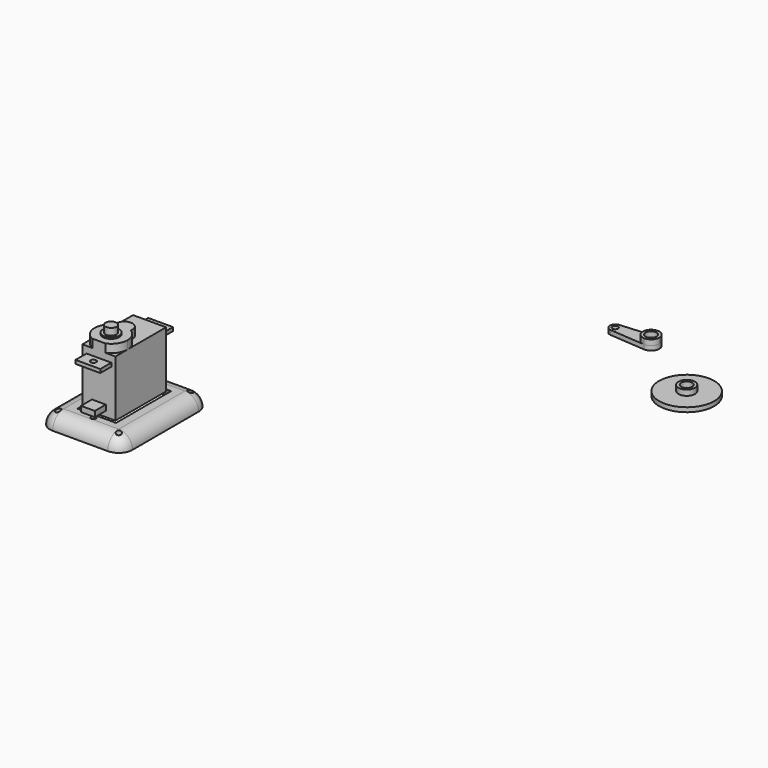
from build123d import *

# Parameters (mm, degrees)
F0_W          = 12
F0_H          = 23
F1_DEPTH      = 20.5
F3_DEPTH      = 3
F4_R          = 3
F5_DEPTH      = 0.5
F6_R          = 2
F7_DEPTH      = 2.5
F9_W          = 9
F9_H          = 5
F9_R          = 1
F10_DEPTH     = 1.3
F11_W         = 5
F11_H         = 2
F12_DEPTH     = 5
F13_R         = 10
F13_R_2       = 2.5
F14_DEPTH     = 0.5
F15_R         = 10
F15_R_2       = 2.5
F15_R_3       = 1
F16_DEPTH     = 1.1
F17_R         = 3
F17_R_2       = 2
F18_DEPTH     = 2
F19_R         = 2.5
F20_DEPTH     = 0.5
F22_R         = 2.5
F22_R_2       = 1
F21_R         = 2.5
F23_DEPTH     = 1.1
F24_R         = 2
F25_DEPTH     = 2
F26_R         = 1.05
F27_DEPTH     = 1.601
F28_W         = 30
F28_H         = 40
F28_R         = 0.9
F28_W_2       = 14
F28_H_2       = 25
F29_DEPTH     = 5
F30_T1_DEPTH  = 20
F30_T3_DEPTH  = 30
F30_T5_DEPTH  = 12.5
F30_S9_W      = 5
F30_S9_H      = 5
F30_T10_DEPTH = 5
F30_S15_W     = 5
F30_S15_H     = 5
F30_T16_DEPTH = 5
F30_S21_W     = 5
F30_S21_H     = 5
F30_T22_DEPTH = 5
F30_S27_W     = 5
F30_S27_H     = 5
F30_T28_DEPTH = 5
F31_T1_DEPTH  = 14


# Not quite as in the source:
# - a fillet or chamfer that OpenCascade refuses, or shapes differently, is made with other operations: its cross-section is extruded or revolved along the edge and cut away or added


with BuildPart() as f1:
    # F0 (on Top) → F1 (new body)
    with BuildSketch(Plane.XY):
        with Locations((-56.6354888082, -51.4608333111)):
            Rectangle(F0_W, F0_H)
    extrude(amount=F1_DEPTH)

    # F2 (on face) → F3 (join)
    with BuildSketch(Plane.XY.offset(20.5)):
        with BuildLine():
            ThreePointArc((-54.2375730465, -62.9608333111), (-51.6161514729, -60.7481198388), (-50.6354888082, -57.4608333111))
            ThreePointArc((-50.6354888082, -57.4608333111), (-51.4669094551, -54.4135743016), (-53.7307512985, -52.2108333111))
            ThreePointArc((-53.7307512985, -52.2108333111), (-56.6354888082, -51.4608333111), (-59.5402263178, -52.2108333111))
            ThreePointArc((-59.5402263178, -52.2108333111), (-61.8040681612, -54.4135743016), (-62.6354888082, -57.4608333111))
            ThreePointArc((-62.6354888082, -57.4608333111), (-61.6548261434, -60.7481198388), (-59.0334045698, -62.9608333111))
            Line((-59.0334045698, -62.9608333111), (-54.2375730465, -62.9608333111))
        make_face()
        with BuildLine():
            ThreePointArc((-59.5402263178, -52.2108333111), (-56.6354888082, -51.4608333111), (-53.7307512985, -52.2108333111))
            ThreePointArc((-53.7307512985, -52.2108333111), (-56.6354888082, -48.4608333111), (-59.5402263178, -52.2108333111))
        make_face()
    extrude(amount=F3_DEPTH)

    # F4 (on face) → F5 (join)
    with BuildSketch(Plane.XY.offset(23.5)):
        with Locations((-56.6354888082, -57.4608333111)):
            Circle(F4_R)
    extrude(amount=F5_DEPTH)

    # F6 (on face) → F7 (join)
    with BuildSketch(Plane.XY.offset(24)):
        with Locations((-56.6354888082, -57.4608333111)):
            Circle(F6_R)
    extrude(amount=F7_DEPTH)

    # F9 (on offset) → F10 (join)
    with BuildSketch(Plane.XY.offset(16.75)):
        with Locations((-56.6354888082, -65.4608333111)):
            Rectangle(F9_W, F9_H)
        with Locations((-56.6354888082, -65.4608333111)):
            Circle(F9_R, mode=Mode.SUBTRACT)
        with Locations((-56.6354888082, -37.4608333111)):
            Rectangle(F9_W, F9_H)
        with Locations((-56.6354888082, -37.4608333111)):
            Circle(F9_R, mode=Mode.SUBTRACT)
    extrude(amount=F10_DEPTH)

    # F11 (on face) → F12 (join, through all)
    with BuildSketch(Plane.XZ.offset(62.9608333111)):
        with Locations((-56.6354888082, 3)):
            Rectangle(F11_W, F11_H)
    extrude(amount=F12_DEPTH)


with BuildPart() as f14:
    # F13 (on Top) → F14 (new body)
    with BuildSketch(Plane.XY):
        with Locations((66.4411634207, 50.0796362758)):
            Circle(F13_R)
        with Locations((66.4411634207, 50.0796362758)):
            Circle(F13_R_2, mode=Mode.SUBTRACT)
    extrude(amount=F14_DEPTH)

    # F15 (on face) → F16 (join)
    with BuildSketch(Plane.XY.offset(0.5)):
        with Locations((66.4411634207, 50.0796362758)):
            Circle(F15_R)
        with Locations((66.4411634207, 50.0796362758)):
            Circle(F15_R_2, mode=Mode.SUBTRACT)
        with Locations((66.4411634207, 50.0796362758)):
            Circle(F15_R_2)
        with Locations((66.4411634207, 50.0796362758)):
            Circle(F15_R_3, mode=Mode.SUBTRACT)
    extrude(amount=F16_DEPTH)

    # F17 (on face) → F18 (join)
    with BuildSketch(Plane.XY.offset(1.6)):
        with Locations((66.4411634207, 50.0796362758)):
            Circle(F17_R)
        with Locations((66.4411634207, 50.0796362758)):
            Circle(F17_R_2, mode=Mode.SUBTRACT)
    extrude(amount=F18_DEPTH)


with BuildPart() as f20:
    # F19 (on Top) → F20 (new body)
    with BuildSketch(Plane.XY):
        with BuildLine():
            Line((26.1375896391, 65.84841691), (39.0606665622, 64.8513798795))
            ThreePointArc((39.0606665622, 64.8513798795), (42.291435793, 67.8424909711), (39.0606665622, 70.8336020627))
            Line((39.0606665622, 70.8336020627), (26.1375896391, 69.8365650321))
            ThreePointArc((26.1375896391, 69.8365650321), (24.291435793, 67.8424909711), (26.1375896391, 65.84841691))
        make_face()
        with Locations((39.291435793, 67.8424909711)):
            Circle(F19_R, mode=Mode.SUBTRACT)
    extrude(amount=F20_DEPTH)

    # F22 (on face) + F21 (on face) → F23 (join)
    with BuildSketch(Plane.XY.offset(0.5)):
        with Locations((39.291435793, 67.8424909711)):
            Circle(F22_R)
        with Locations((39.291435793, 67.8424909711)):
            Circle(F22_R_2, mode=Mode.SUBTRACT)
    with BuildSketch(Plane.XY.offset(0.5)):
        with BuildLine():
            ThreePointArc((39.0606665622, 64.8513798795), (42.291435793, 67.8424909711), (39.0606665622, 70.8336020627))
            Line((39.0606665622, 70.8336020627), (26.1375896391, 69.8365650321))
            ThreePointArc((26.1375896391, 69.8365650321), (24.291435793, 67.8424909711), (26.1375896391, 65.84841691))
            Line((26.1375896391, 65.84841691), (39.0606665622, 64.8513798795))
        make_face()
        with Locations((39.291435793, 67.8424909711)):
            Circle(F21_R, mode=Mode.SUBTRACT)
    extrude(amount=F23_DEPTH)

    # F24 (on face) → F25 (join)
    with BuildSketch(Plane.XY.offset(1.6)):
        with BuildLine():
            ThreePointArc((39.0606665622, 64.8513798795), (41.3295344544, 65.641092814), (42.291435793, 67.8424909711))
            ThreePointArc((42.291435793, 67.8424909711), (41.3295344544, 70.0438891282), (39.0606665622, 70.8336020627))
            ThreePointArc((39.0606665622, 70.8336020627), (36.291435793, 67.8424909711), (39.0606665622, 64.8513798795))
        make_face()
        with Locations((39.291435793, 67.8424909711)):
            Circle(F24_R, mode=Mode.SUBTRACT)
    extrude(amount=F25_DEPTH)

    # F26 (on face) → F27 (cut, through all)
    with BuildSketch(Plane.XY.offset(1.6)):
        with Locations((26.291435793, 67.8424909711)):
            Circle(F26_R)
    extrude(amount=-F27_DEPTH, mode=Mode.SUBTRACT)


with BuildPart() as f29:
    # F28 (on face) → F29 (new body)
    with BuildSketch(Plane(origin=(0, 0, 0), x_dir=(1, 0, 0), z_dir=(0, 0, -1))):
        with Locations((-56.6354888082, 51.4608333111)):
            Rectangle(F28_W, F28_H)
        with Locations((-67.6354888082, 35.2108333111)):
            Circle(F28_R, mode=Mode.SUBTRACT)
        with Locations((-56.6354888082, 37.4608333111)):
            Circle(F28_R, mode=Mode.SUBTRACT)
        with Locations((-45.6354888082, 35.2108333111)):
            Circle(F28_R, mode=Mode.SUBTRACT)
        with Locations((-56.6354888082, 51.4608333111)):
            Rectangle(F28_W_2, F28_H_2, mode=Mode.SUBTRACT)
        with Locations((-67.6354888082, 67.7108333111)):
            Circle(F28_R, mode=Mode.SUBTRACT)
        with Locations((-56.6354888082, 65.4608333111)):
            Circle(F28_R, mode=Mode.SUBTRACT)
        with Locations((-45.6354888082, 67.7108333111)):
            Circle(F28_R, mode=Mode.SUBTRACT)
    extrude(amount=F29_DEPTH)

    # F30: fillet of radius 5 on 8 edges, made by hand

    # F30_s2 → F30_t1 (cut)
    with BuildSketch(Plane.YZ.offset(-66.6354888082)):
        with BuildLine():
            ThreePointArc((-71.4608333111, -5), (-69.996367217, -1.4644660941), (-66.4608333111, 0))
            Line((-66.4608333111, 0), (-71.4608333111, 0))
            Line((-71.4608333111, 0), (-71.4608333111, -5))
        make_face()
        with BuildLine():
            ThreePointArc((-31.4608333111, -5), (-32.9252994051, -1.4644660941), (-36.4608333111, 0))
            Line((-36.4608333111, 0), (-31.4608333111, 0))
            Line((-31.4608333111, 0), (-31.4608333111, -5))
        make_face()
    extrude(amount=F30_T1_DEPTH, mode=Mode.SUBTRACT)

    # F30_s4 → F30_t3 (cut)
    with BuildSketch(Plane.XZ.offset(36.4608333111)):
        with BuildLine():
            ThreePointArc((-71.6354888082, -5), (-70.1710227141, -1.4644660941), (-66.6354888082, 0))
            Line((-66.6354888082, 0), (-71.6354888082, 0))
            Line((-71.6354888082, 0), (-71.6354888082, -5))
        make_face()
        with BuildLine():
            ThreePointArc((-41.6354888082, -5), (-43.0999549022, -1.4644660941), (-46.6354888082, 0))
            Line((-46.6354888082, 0), (-41.6354888082, 0))
            Line((-41.6354888082, 0), (-41.6354888082, -5))
        make_face()
    extrude(amount=F30_T3_DEPTH, mode=Mode.SUBTRACT)

    # F30_s6 → F30_t5 (cut)
    with BuildSketch(Plane.XY.offset(-17.5)):
        with BuildLine():
            ThreePointArc((-66.6354888082, -71.4608333111), (-70.1710227141, -69.996367217), (-71.6354888082, -66.4608333111))
            Line((-71.6354888082, -66.4608333111), (-71.6354888082, -71.4608333111))
            Line((-71.6354888082, -71.4608333111), (-66.6354888082, -71.4608333111))
        make_face()
        with BuildLine():
            ThreePointArc((-46.6354888082, -71.4608333111), (-43.0999549022, -69.996367217), (-41.6354888082, -66.4608333111))
            Line((-41.6354888082, -66.4608333111), (-41.6354888082, -71.4608333111))
            Line((-41.6354888082, -71.4608333111), (-46.6354888082, -71.4608333111))
        make_face()
        with BuildLine():
            ThreePointArc((-46.6354888082, -31.4608333111), (-43.0999549022, -32.9252994051), (-41.6354888082, -36.4608333111))
            Line((-41.6354888082, -36.4608333111), (-41.6354888082, -31.4608333111))
            Line((-41.6354888082, -31.4608333111), (-46.6354888082, -31.4608333111))
        make_face()
        with BuildLine():
            ThreePointArc((-71.6354888082, -36.4608333111), (-70.1710227141, -32.9252994051), (-66.6354888082, -31.4608333111))
            Line((-66.6354888082, -31.4608333111), (-71.6354888082, -31.4608333111))
            Line((-71.6354888082, -31.4608333111), (-71.6354888082, -36.4608333111))
        make_face()
    extrude(amount=F30_T5_DEPTH, mode=Mode.SUBTRACT)


with BuildPart() as f30_tool8:
    # F30_s9 → F30_t10 (new body)
    with BuildSketch(Plane.XZ.offset(66.4608333111)):
        with Locations((-44.1354888082, -2.5)):
            Rectangle(F30_S9_W, F30_S9_H)
    extrude(amount=F30_T10_DEPTH)

    # F30_s11 → F30_t12 (revolve, cut)
    with BuildSketch(Plane(origin=(-46.6354888082, -66.4608333111, -5), x_dir=(-0.7071067812, 0, -0.7071067812), z_dir=(-0.7071067812, 0, 0.7071067812))):
        with BuildLine():
            ThreePointArc((0, -5), (5, 0), (0, 5))
            Line((0, 5), (0, -5))
        make_face()
    revolve(axis=Axis((-46.6354888082, -66.4608333111, -5), (0, -1, 0)), mode=Mode.SUBTRACT)


with BuildPart() as f29_1:
    add(f29.part)

    # F30_t7: cut F30_tool8
    add(f30_tool8.part, mode=Mode.SUBTRACT)


with BuildPart() as f30_tool14:
    # F30_s15 → F30_t16 (new body)
    with BuildSketch(Plane.XZ.offset(66.4608333111)):
        with Locations((-69.1354888082, -2.5)):
            Rectangle(F30_S15_W, F30_S15_H)
    extrude(amount=F30_T16_DEPTH)

    # F30_s17 → F30_t18 (revolve, cut)
    with BuildSketch(Plane(origin=(-66.6354888082, -66.4608333111, -5), x_dir=(0.7071067812, 0, -0.7071067812), z_dir=(-0.7071067812, 0, -0.7071067812))):
        with BuildLine():
            ThreePointArc((0, -5), (5, 0), (0, 5))
            Line((0, 5), (0, -5))
        make_face()
    revolve(axis=Axis((-66.6354888082, -66.4608333111, -5), (0, -1, 0)), mode=Mode.SUBTRACT)


with BuildPart() as f29_2:
    add(f29_1.part)

    # F30_t13: cut F30_tool14
    add(f30_tool14.part, mode=Mode.SUBTRACT)


with BuildPart() as f30_tool20:
    # F30_s21 → F30_t22 (new body)
    with BuildSketch(Plane.YZ.offset(-66.6354888082)):
        with Locations((-33.9608333111, -2.5)):
            Rectangle(F30_S21_W, F30_S21_H)
    extrude(amount=-F30_T22_DEPTH)

    # F30_s23 → F30_t24 (revolve, cut)
    with BuildSketch(Plane(origin=(-66.6354888082, -36.4608333111, -5), x_dir=(0, -0.7071067812, -0.7071067812), z_dir=(0, 0.7071067812, -0.7071067812))):
        with BuildLine():
            ThreePointArc((0, -5), (5, 0), (0, 5))
            Line((0, 5), (0, -5))
        make_face()
    revolve(axis=Axis((-66.6354888082, -36.4608333111, -5), (-1, 0, 0)), mode=Mode.SUBTRACT)


with BuildPart() as f29_3:
    add(f29_2.part)

    # F30_t19: cut F30_tool20
    add(f30_tool20.part, mode=Mode.SUBTRACT)


with BuildPart() as f30_tool26:
    # F30_s27 → F30_t28 (new body)
    with BuildSketch(Plane.XZ.offset(36.4608333111)):
        with Locations((-44.1354888082, -2.5)):
            Rectangle(F30_S27_W, F30_S27_H)
    extrude(amount=-F30_T28_DEPTH)

    # F30_s29 → F30_t30 (revolve, cut)
    with BuildSketch(Plane(origin=(-46.6354888082, -36.4608333111, -5), x_dir=(-0.7071067812, 0, -0.7071067812), z_dir=(0.7071067812, 0, -0.7071067812))):
        with BuildLine():
            ThreePointArc((0, -5), (5, 0), (0, 5))
            Line((0, 5), (0, -5))
        make_face()
    revolve(axis=Axis((-46.6354888082, -36.4608333111, -5), (0, 1, 0)), mode=Mode.SUBTRACT)


with BuildPart() as f29_4:
    add(f29_3.part)

    # F30_t25: cut F30_tool26
    add(f30_tool26.part, mode=Mode.SUBTRACT)

    # F31: fillet of radius 7 on 2 edges, made by hand

    # F31_s2 → F31_t1 (cut)
    with BuildSketch(Plane.YZ.offset(-63.6354888082)):
        with BuildLine():
            ThreePointArc((-70.6690372436, -5), (-66.4857371109, -3.6124860802), (-63.9608333111, 0))
            Line((-63.9608333111, 0), (-63.9608333111, -5))
            Line((-63.9608333111, -5), (-70.6690372436, -5))
        make_face()
        with BuildLine():
            ThreePointArc((-32.2526293786, -5), (-36.4359295113, -3.6124860802), (-38.9608333111, 0))
            Line((-38.9608333111, 0), (-38.9608333111, -5))
            Line((-38.9608333111, -5), (-32.2526293786, -5))
        make_face()
    extrude(amount=F31_T1_DEPTH, mode=Mode.SUBTRACT)


solid = Compound([f1.part, f14.part, f20.part, f29_4.part])
